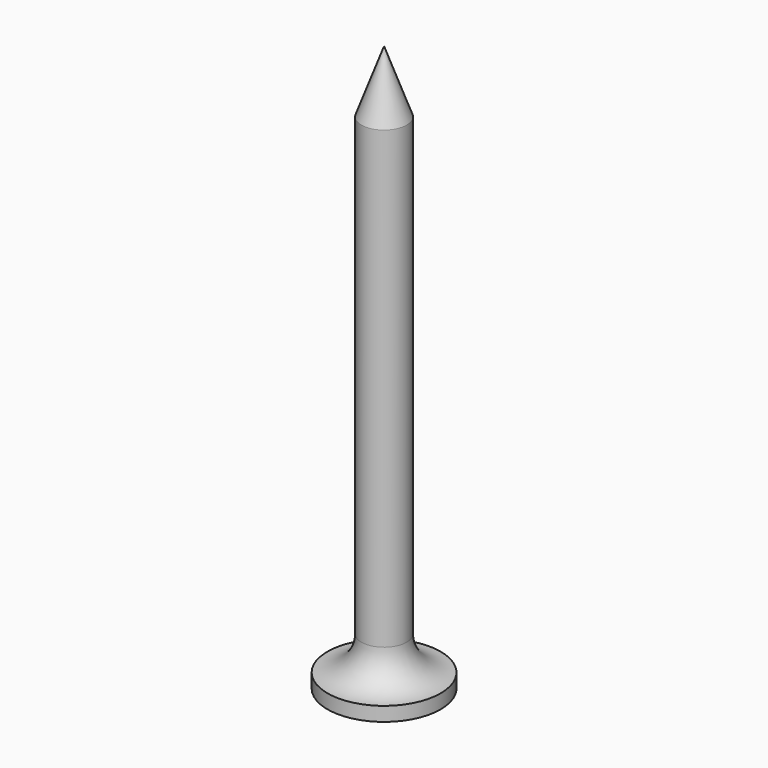
from build123d import *

# Parameters (mm, degrees)
F3_DEPTH        = 1
F3_COPIES_COUNT = 4


# Not quite as in the source:
# - a pattern or mirror of a feature is missing from the dataset's text; its kind, count and spacing are read off the source's solid


with BuildPart() as f1:
    # F0 (on Front) → F1 (revolve)
    with BuildSketch(Plane.XZ):
        with BuildLine():
            Line((1.6, 35.6040361289), (0, 40))
            Line((0, 40), (0, 0))
            Line((0, 0), (4, 0))
            Line((4, 0), (4, 1))
            ThreePointArc((4, 1), (2.3029437252, 1.7029437252), (1.6, 3.4))
            Line((1.6, 3.4), (1.6, 35.6040361289))
        make_face()
    revolve(axis=Axis((0, 0, 20), (0, 0, 1)))

    # F2 (on Top) → F3 (cut)
    with BuildSketch(Plane.XY):
        Polygon((2.5, 0), (0, 0), (0, -2.5), (0.5, -2.5), (0.5, -0.5), (2.5, -0.5), align=None)
    f3 = extrude(amount=F3_DEPTH, mode=Mode.SUBTRACT)

    # F3_copies: F3 ×4 about axis
    f3_copies_axis = Axis((0, 0, 0), (0, 0, 1))
    for i in range(1, F3_COPIES_COUNT):
        add(f3.rotate(f3_copies_axis, i * 360 / F3_COPIES_COUNT), mode=Mode.SUBTRACT)


solid = f1.part
